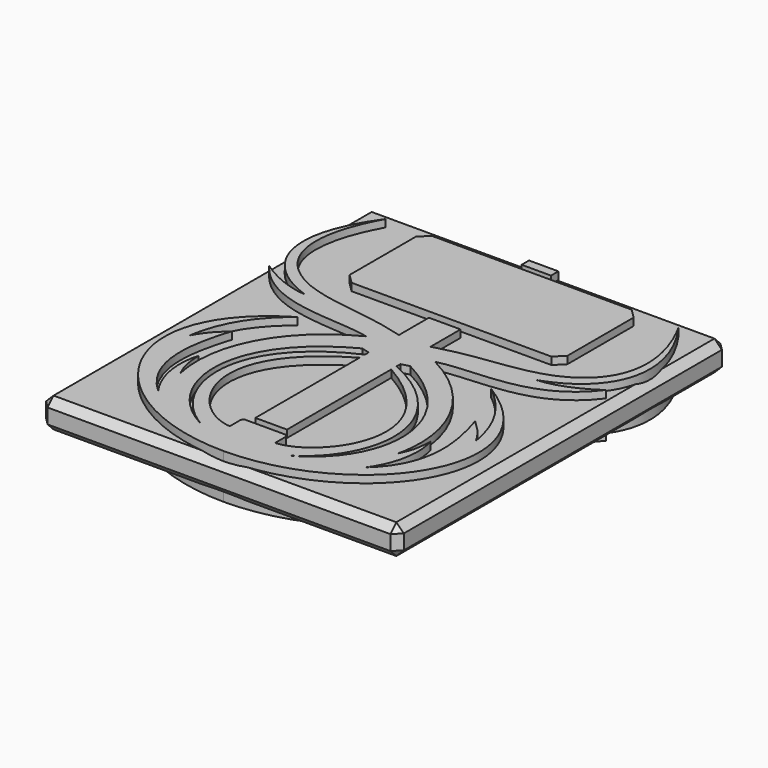
from build123d import *

# Parameters (mm, degrees)
F1_DEPTH     = 6.35
F2_DEPTH     = 9.525
F3_T1_DEPTH  = 4.0327916303
F3_T3_DEPTH  = 4.0327916303
F3_T5_DEPTH  = 4.0327916303
F3_T7_DEPTH  = 4.0327916303
F3_T9_DEPTH  = 4.0327916303
F3_T11_DEPTH = 4.0327916303
F3_T13_DEPTH = 4.0327916303
F3_T15_DEPTH = 4.0327916303
F3_T17_DEPTH = 29.0301869736
F3_T19_DEPTH = 192.1295719037
F3_T21_DEPTH = 168.7301869736


# Not quite as in the source:
# - a fillet or chamfer that OpenCascade refuses, or shapes differently, is made with other operations: its cross-section is extruded or revolved along the edge and cut away or added


with BuildPart() as f1:
    # F0 (on Top) → F1 (new body, symmetric)
    with BuildSketch(Plane.XY):
        Polygon((-76.3395167732, -75.9592950344), (-0.1395167732, -75.9592950344), (76.0604832268, -75.9592950344), (76.0604832268, 99.8400898957), (-0.3772020667, 99.8400898957), (-76.3395167732, 99.8400898957), align=None)
        with BuildLine():
            Line((-6.8799913861, 44.2892052233), (-0.1395167732, 44.2892052233))
            Line((-0.1395167732, 44.2892052233), (6.6009578396, 44.2892052233))
            Line((6.6009578396, 44.2892052233), (6.6009578396, 28.3039733768))
            add(Edge.make_bspline(
                [(6.6009578396, 28.3039733768), (26.5900306505, 33.9711308479), (37.0916825043, 32.1136220375), (51.7776187764, 37.7081698754)],
                knots=[0, 0, 0, 0, 46.1450929697, 46.1450929697, 46.1450929697, 46.1450929697], degree=3))
            add(Edge.make_bspline(
                [(51.7776187764, 37.7081698754), (73.0898510766, 46.7012859881), (75.5619611692, 66.6821375489), (62.3242836547, 90.7550230622)],
                knots=[0, 0, 0, 0, 54.0851252479, 54.0851252479, 54.0851252479, 54.0851252479], degree=3))
            add(Edge.make_bspline(
                [(62.3242836547, 90.7550230622), (70.2098065026, 79.8010850957), (73.6896972191, 69.8762632372), (73.6896974189, 61.3201553811)],
                knots=[0, 0, 0, 0, 22.7856930091, 22.7856930091, 22.7856930091, 22.7856930091], degree=3))
            add(Edge.make_bspline(
                [(73.6896974189, 61.3201553811), (73.6896977509, 47.1026080353), (64.0810465009, 36.6643450953), (49.1112602689, 31.5635202295)],
                knots=[22.7856930091, 22.7856930091, 22.7856930091, 22.7856930091, 60.6483140293, 60.6483140293, 60.6483140293, 60.6483140293], degree=3))
            add(Edge.make_bspline(
                [(49.1112602689, 31.5635202295), (56.512868042, 32.0529900491), (64.7170897674, 35.515807569), (71.6427248072, 40.4170304537)],
                knots=[0, 0, 0, 0, 24.2085013484, 24.2085013484, 24.2085013484, 24.2085013484], degree=3))
            add(Edge.make_bspline(
                [(71.6427248072, 40.4170304537), (55.7588432085, 19.1547237337), (30.2959364009, 24.5825536549), (14.5286014405, 20.7954701036)],
                knots=[0, 0, 0, 0, 60.390634361, 60.390634361, 60.390634361, 60.390634361], degree=3))
            add(Edge.make_bspline(
                [(14.5286014405, 20.7954701036), (41.5803175521, 6.7990645766), (51.0726925087, -18.260801211), (46.0924860191, -38.8492196798)],
                knots=[0, 0, 0, 0, 67.4816110437, 67.4816110437, 67.4816110437, 67.4816110437], degree=3))
            add(Edge.make_bspline(
                [(46.0924860191, -38.8492196798), (48.3534094047, -34.169908613), (49.0401517701, -31.6784828901), (49.3026469004, -25.0572301447)],
                knots=[0, 0, 0, 0, 14.1606535238, 14.1606535238, 14.1606535238, 14.1606535238], degree=3))
            add(Edge.make_bspline(
                [(49.3026469004, -25.0572301447), (51.7310705137, -32.9342447221), (50.7265012812, -43.7572076917), (44.0818425369, -53.0597306788)],
                knots=[0, 0, 0, 0, 28.4850282493, 28.4850282493, 28.4850282493, 28.4850282493], degree=3))
            add(Edge.make_bspline(
                [(44.0818425369, -53.0597306788), (60.305254544, -38.450088352), (56.4526263725, -19.4557197392), (51.6902711343, -4.2840936221)],
                knots=[0, 0, 0, 0, 49.3654834475, 49.3654834475, 49.3654834475, 49.3654834475], degree=3))
            add(Edge.make_bspline(
                [(51.6902711343, -4.2840936221), (54.9464095485, -7.2530964389), (58.2408178699, -10.4841506109), (60.8383324098, -15.4891163111)],
                knots=[0, 0, 0, 0, 14.465115228, 14.465115228, 14.465115228, 14.465115228], degree=3))
            add(Edge.make_bspline(
                [(60.8383324098, -15.4891163111), (58.5245881331, -1.1494335486), (51.5281986546, 9.0760597959), (41.0085301947, 17.3916071653)],
                knots=[0, 0, 0, 0, 38.3974352297, 38.3974352297, 38.3974352297, 38.3974352297], degree=3))
            add(Edge.make_bspline(
                [(41.0085301947, 17.3916071653), (94.1427406025, -14.5556982607), (57.5462374937, -73.1422898984), (-0.1395167732, -73.4192950344)],
                knots=[0, 0, 0, 0, 99.6984539881, 99.6984539881, 99.6984539881, 99.6984539881], degree=3))
            add(Edge.make_bspline(
                [(-41.2875637412, 17.3916071653), (-94.4217741489, -14.5556982607), (-57.8252710402, -73.1422898984), (-0.1395167732, -73.4192950344)],
                knots=[0, 0, 0, 0, 99.6984539881, 99.6984539881, 99.6984539881, 99.6984539881], degree=3))
            add(Edge.make_bspline(
                [(-61.1173659563, -15.4891163111), (-58.8036216795, -1.1494335486), (-51.8072322011, 9.0760597959), (-41.2875637412, 17.3916071653)],
                knots=[0, 0, 0, 0, 38.3974352297, 38.3974352297, 38.3974352297, 38.3974352297], degree=3))
            add(Edge.make_bspline(
                [(-51.9693046808, -4.2840936221), (-55.225443095, -7.2530964389), (-58.5198514163, -10.4841506109), (-61.1173659563, -15.4891163111)],
                knots=[0, 0, 0, 0, 14.465115228, 14.465115228, 14.465115228, 14.465115228], degree=3))
            add(Edge.make_bspline(
                [(-44.3608760834, -53.0597306788), (-60.5842880905, -38.450088352), (-56.731659919, -19.4557197392), (-51.9693046808, -4.2840936221)],
                knots=[0, 0, 0, 0, 49.3654834475, 49.3654834475, 49.3654834475, 49.3654834475], degree=3))
            add(Edge.make_bspline(
                [(-49.5816804469, -25.0572301447), (-52.0101040602, -32.9342447221), (-51.0055348277, -43.7572076917), (-44.3608760834, -53.0597306788)],
                knots=[0, 0, 0, 0, 28.4850282493, 28.4850282493, 28.4850282493, 28.4850282493], degree=3))
            add(Edge.make_bspline(
                [(-46.3715195656, -38.8492196798), (-48.6324429512, -34.169908613), (-49.3191853166, -31.6784828901), (-49.5816804469, -25.0572301447)],
                knots=[0, 0, 0, 0, 14.1606535238, 14.1606535238, 14.1606535238, 14.1606535238], degree=3))
            add(Edge.make_bspline(
                [(-14.8076349869, 20.7954701036), (-41.8593510985, 6.7990645766), (-51.3517260551, -18.260801211), (-46.3715195656, -38.8492196798)],
                knots=[0, 0, 0, 0, 67.4816110437, 67.4816110437, 67.4816110437, 67.4816110437], degree=3))
            add(Edge.make_bspline(
                [(-71.9217583537, 40.4170304537), (-56.037876755, 19.1547237337), (-30.5749699473, 24.5825536549), (-14.8076349869, 20.7954701036)],
                knots=[0, 0, 0, 0, 60.390634361, 60.390634361, 60.390634361, 60.390634361], degree=3))
            add(Edge.make_bspline(
                [(-49.3902938154, 31.5635202295), (-56.7919015884, 32.0529900491), (-64.9961233139, 35.515807569), (-71.9217583537, 40.4170304537)],
                knots=[0, 0, 0, 0, 24.2085013484, 24.2085013484, 24.2085013484, 24.2085013484], degree=3))
            add(Edge.make_bspline(
                [(-73.9687309654, 61.3201553811), (-73.9687312974, 47.1026080353), (-64.3600800474, 36.6643450953), (-49.3902938154, 31.5635202295)],
                knots=[22.7856930091, 22.7856930091, 22.7856930091, 22.7856930091, 60.6483140293, 60.6483140293, 60.6483140293, 60.6483140293], degree=3))
            add(Edge.make_bspline(
                [(-62.6033172011, 90.7550230622), (-70.4888400491, 79.8010850957), (-73.9687307656, 69.8762632372), (-73.9687309654, 61.3201553811)],
                knots=[0, 0, 0, 0, 22.7856930091, 22.7856930091, 22.7856930091, 22.7856930091], degree=3))
            add(Edge.make_bspline(
                [(-52.0566523229, 37.7081698754), (-73.3688846231, 46.7012859881), (-75.8409947157, 66.6821375489), (-62.6033172011, 90.7550230622)],
                knots=[0, 0, 0, 0, 54.0851252479, 54.0851252479, 54.0851252479, 54.0851252479], degree=3))
            add(Edge.make_bspline(
                [(-6.8799913861, 28.3039733768), (-26.8690641969, 33.9711308479), (-37.3707160507, 32.1136220375), (-52.0566523229, 37.7081698754)],
                knots=[0, 0, 0, 0, 46.1450929697, 46.1450929697, 46.1450929697, 46.1450929697], degree=3))
            Line((-6.8799913861, 28.3039733768), (-6.8799913861, 44.2892052233))
        make_face(mode=Mode.SUBTRACT)
        Polygon((-46.7502180452, 87.1615596313), (-42.9751879819, 90.9365896945), (42.2207838486, 90.9365896945), (46.2334992052, 86.9238743379), (46.2334992052, 51.6543717875), (42.458469142, 47.8793417243), (-42.7375026885, 47.8793417243), (-46.7502180452, 51.892057081), align=None, mode=Mode.SUBTRACT)
        Polygon((-6.6463192925, 97.3000898957), (-0.3772020667, 97.3000898957), (5.8919151591, 97.3000898957), (5.8919151591, 93.3534055948), (-0.3772020667, 93.3534055948), (-6.6463192925, 93.3534055948), align=None, mode=Mode.SUBTRACT)
    extrude(amount=F1_DEPTH, both=True)

    # F3: chamfer of 3.175 on 12 edges, made by hand

    # F3_s2 → F3_t1 (cut)
    with BuildSketch(Plane(origin=(50.6732594204, -50.6732594204, -50.6732594204), x_dir=(0.7071067812, 0.7071067812, 0), z_dir=(0.5773502692, -0.5773502692, -0.5773502692))):
        Polygon((0.071550857, 54.2846846585), (2.3166148873, 58.1732496251), (-2.1735131733, 58.1732496251), align=None)
    extrude(amount=F3_T1_DEPTH, mode=Mode.SUBTRACT)

    # F3_s4 → F3_t3 (cut)
    with BuildSketch(Plane(origin=(50.6732594204, -50.6732594204, 50.6732594204), x_dir=(0.7071067812, 0.7071067812, 0), z_dir=(0.5773502692, -0.5773502692, 0.5773502692))):
        Polygon((2.3166148873, -58.1732496251), (0.071550857, -54.2846846585), (-2.1735131733, -58.1732496251), align=None)
    extrude(amount=F3_T3_DEPTH, mode=Mode.SUBTRACT)

    # F3_s6 → F3_t5 (cut)
    with BuildSketch(Plane(origin=(58.6335243742, 58.6335243742, -58.6335243742), x_dir=(-0.7071067812, 0.7071067812, 0), z_dir=(0.5773502692, 0.5773502692, -0.5773502692))):
        Polygon((16.8147211296, 64.0339783355), (19.0597851598, 67.9225433022), (14.5696570993, 67.9225433022), align=None)
    extrude(amount=F3_T5_DEPTH, mode=Mode.SUBTRACT)

    # F3_s8 → F3_t7 (cut)
    with BuildSketch(Plane(origin=(58.6335243742, 58.6335243742, 58.6335243742), x_dir=(-0.7071067812, 0.7071067812, 0), z_dir=(0.5773502692, 0.5773502692, 0.5773502692))):
        Polygon((19.0597851598, -67.9225433022), (14.5696570993, -67.9225433022), (16.8147211296, -64.0339783355), align=None)
    extrude(amount=F3_T7_DEPTH, mode=Mode.SUBTRACT)

    # F3_s10 → F3_t9 (cut)
    with BuildSketch(Plane(origin=(-58.7265355563, 58.7265355563, -58.7265355563), x_dir=(-0.7071067812, -0.7071067812, 0), z_dir=(-0.5773502692, 0.5773502692, -0.5773502692))):
        Polygon((-14.3723505864, 68.0364582705), (-18.8624786469, 68.0364582705), (-16.6174146167, 64.1478933039), align=None)
    extrude(amount=F3_T9_DEPTH, mode=Mode.SUBTRACT)

    # F3_s12 → F3_t11 (cut)
    with BuildSketch(Plane(origin=(-50.7662706026, -50.7662706026, -50.7662706026), x_dir=(0.7071067812, -0.7071067812, 0), z_dir=(-0.5773502692, -0.5773502692, -0.5773502692))):
        Polygon((-2.5139214002, 58.2871645935), (-0.2688573699, 54.3985996268), (1.9762066604, 58.2871645935), align=None)
    extrude(amount=F3_T11_DEPTH, mode=Mode.SUBTRACT)

    # F3_s14 → F3_t13 (cut)
    with BuildSketch(Plane(origin=(-50.7662706026, -50.7662706026, 50.7662706026), x_dir=(0.7071067812, -0.7071067812, 0), z_dir=(-0.5773502692, -0.5773502692, 0.5773502692))):
        Polygon((-2.5139214002, -58.2871645935), (-0.2688573699, -54.3985996268), (1.9762066604, -58.2871645935), align=None)
    extrude(amount=F3_T13_DEPTH, mode=Mode.SUBTRACT)

    # F3_s16 → F3_t15 (cut)
    with BuildSketch(Plane(origin=(-58.7265355563, 58.7265355563, 58.7265355563), x_dir=(-0.7071067812, -0.7071067812, 0), z_dir=(-0.5773502692, 0.5773502692, 0.5773502692))):
        Polygon((-14.3723505864, -68.0364582705), (-18.8624786469, -68.0364582705), (-16.6174146167, -64.1478933039), align=None)
    extrude(amount=F3_T15_DEPTH, mode=Mode.SUBTRACT)

    # F3_s18 → F3_t17 (cut)
    with BuildSketch(Plane.XY.offset(-14.5150934868)):
        Polygon((76.0604832268, -72.7842950344), (72.8854832268, -75.9592950344), (76.0604832268, -75.9592950344), align=None)
        Polygon((72.8854832268, 99.8400898957), (76.0604832268, 96.6650898957), (76.0604832268, 99.8400898957), align=None)
        Polygon((-76.3395167732, -72.7842950344), (-73.1645167732, -75.9592950344), (-76.3395167732, -75.9592950344), align=None)
        Polygon((-76.3395167732, 96.6650898957), (-73.1645167732, 99.8400898957), (-76.3395167732, 99.8400898957), align=None)
    extrude(amount=F3_T17_DEPTH, mode=Mode.SUBTRACT)

    # F3_s20 → F3_t19 (cut)
    with BuildSketch(Plane.XZ.offset(-108.0051833825)):
        Polygon((76.0604832268, -3.175), (72.8854832268, -6.35), (76.0604832268, -6.35), align=None)
        Polygon((76.0604832268, 3.175), (72.8854832268, 6.35), (76.0604832268, 6.35), align=None)
        Polygon((-76.3395167732, -3.175), (-73.1645167732, -6.35), (-76.3395167732, -6.35), align=None)
        Polygon((-76.3395167732, 3.175), (-73.1645167732, 6.35), (-76.3395167732, 6.35), align=None)
    extrude(amount=F3_T19_DEPTH, mode=Mode.SUBTRACT)

    # F3_s22 → F3_t21 (cut)
    with BuildSketch(Plane.YZ.offset(-84.50461026)):
        Polygon((99.8400898957, 3.175), (96.6650898957, 6.35), (99.8400898957, 6.35), align=None)
        Polygon((99.8400898957, -3.175), (96.6650898957, -6.35), (99.8400898957, -6.35), align=None)
        Polygon((-75.9592950344, -3.175), (-72.7842950344, -6.35), (-75.9592950344, -6.35), align=None)
        Polygon((-72.7842950344, 6.35), (-75.9592950344, 3.175), (-75.9592950344, 6.35), align=None)
    extrude(amount=F3_T21_DEPTH, mode=Mode.SUBTRACT)


with BuildPart() as f1b:
    # F0 (on Top) → F1, piece 2 (new body, symmetric)
    with BuildSketch(Plane.XY):
        with BuildLine():
            Line((10.0785959613, 13.1602436304), (6.6009578396, 12.2357811779))
            Line((6.6009578396, 12.2357811779), (6.6009578396, 10.2524096146))
            add(Edge.make_bspline(
                [(6.6009578396, 10.2524096146), (49.2393244159, -9.3698259443), (42.5547603619, -48.4816730022), (18.2863567125, -62.6636892557)],
                knots=[0, 0, 0, 0, 73.8465031081, 73.8465031081, 73.8465031081, 73.8465031081], degree=3))
            add(Edge.make_bspline(
                [(10.0785959613, 13.1602436304), (50.5656320703, -8.0102328211), (46.5370509874, -48.0550006032), (18.2863567125, -62.6636892557)],
                knots=[0, 0, 0, 0, 76.266874427, 76.266874427, 76.266874427, 76.266874427], degree=3))
        make_face()
    extrude(amount=F1_DEPTH, both=True)


with BuildPart() as f1c:
    # F0 (on Top) → F1, piece 3 (new body, symmetric)
    with BuildSketch(Plane.XY):
        with BuildLine():
            Line((-6.8799913861, 10.2524096146), (-6.8799913861, 12.2357811779))
            Line((-6.8799913861, 12.2357811779), (-10.3576295078, 13.1602436304))
            add(Edge.make_bspline(
                [(-10.3576295078, 13.1602436304), (-50.8446656168, -8.0102328211), (-46.8160845339, -48.0550006032), (-18.565390259, -62.6636892557)],
                knots=[0, 0, 0, 0, 76.266874427, 76.266874427, 76.266874427, 76.266874427], degree=3))
            add(Edge.make_bspline(
                [(-6.8799913861, 10.2524096146), (-49.5183579624, -9.3698259443), (-42.8337939084, -48.4816730022), (-18.565390259, -62.6636892557)],
                knots=[0, 0, 0, 0, 73.8465031081, 73.8465031081, 73.8465031081, 73.8465031081], degree=3))
        make_face()
    extrude(amount=F1_DEPTH, both=True)


with BuildPart() as f1d:
    # F0 (on Top) → F1, piece 4 (new body, symmetric)
    with BuildSketch(Plane.XY):
        with BuildLine():
            Line((-6.8799913861, -48.1430366635), (-6.8799913861, 7.4029280804))
            add(Edge.make_bspline(
                [(-6.8799913861, 7.4029280804), (-54.2476996779, -19.9007634073), (-27.8019402176, -56.9516755641), (-9.7830155864, -58.1491813064)],
                knots=[0, 0, 0, 0, 65.6163591992, 65.6163591992, 65.6163591992, 65.6163591992], degree=3))
            Line((-9.7830155864, -58.1491813064), (-9.7830155864, -52.2294081748))
            Line((-9.7830155864, -52.2294081748), (-8.9240176603, -51.2886494398))
            Line((-8.9240176603, -51.2886494398), (-0.1395167732, -51.2886494398))
            Line((-0.1395167732, -51.2886494398), (8.6449841138, -51.2886494398))
            Line((8.6449841138, -51.2886494398), (9.5039820399, -52.2294081748))
            Line((9.5039820399, -52.2294081748), (9.5039820399, -58.1491813064))
            add(Edge.make_bspline(
                [(6.6009578396, 7.4029280804), (53.9686661315, -19.9007634073), (27.5229066711, -56.9516755641), (9.5039820399, -58.1491813064)],
                knots=[0, 0, 0, 0, 65.6163591992, 65.6163591992, 65.6163591992, 65.6163591992], degree=3))
            Line((6.6009578396, 7.4029280804), (6.6009578396, -48.1430366635))
            Line((6.6009578396, -48.1430366635), (-0.1395167732, -48.1430366635))
            Line((-0.1395167732, -48.1430366635), (-6.8799913861, -48.1430366635))
        make_face()
    extrude(amount=F1_DEPTH, both=True)


with BuildPart() as f2:
    # F0 (on Top) → F2 (new body, symmetric)
    with BuildSketch(Plane.XY):
        Polygon((42.2207838486, 90.9365896945), (-42.9751879819, 90.9365896945), (-46.7502180452, 87.1615596313), (-46.7502180452, 51.892057081), (-42.7375026885, 47.8793417243), (42.458469142, 47.8793417243), (46.2334992052, 51.6543717875), (46.2334992052, 86.9238743379), align=None)
    extrude(amount=F2_DEPTH, both=True)


with BuildPart() as f2b:
    # F0 (on Top) → F2, piece 2 (new body, symmetric)
    with BuildSketch(Plane.XY):
        Polygon((5.8919151591, 97.3000898957), (-0.3772020667, 97.3000898957), (-6.6463192925, 97.3000898957), (-6.6463192925, 93.3534055948), (-0.3772020667, 93.3534055948), (5.8919151591, 93.3534055948), align=None)
    extrude(amount=F2_DEPTH, both=True)


with BuildPart() as f2c:
    # F0 (on Top) → F2, piece 3 (new body, symmetric)
    with BuildSketch(Plane.XY):
        Polygon((6.6009578396, 44.2892052233), (-0.1395167732, 44.2892052233), (-6.8799913861, 44.2892052233), (-6.8799913861, 28.3039733768), (-6.8799913861, 12.2357811779), (-6.8799913861, 10.2524096146), (-6.8799913861, 7.4029280804), (-6.8799913861, -48.1430366635), (-0.1395167732, -48.1430366635), (6.6009578396, -48.1430366635), (6.6009578396, 7.4029280804), (6.6009578396, 10.2524096146), (6.6009578396, 12.2357811779), (6.6009578396, 28.3039733768), align=None)
        with BuildLine():
            Line((-6.8799913861, 12.2357811779), (-6.8799913861, 28.3039733768))
            add(Edge.make_bspline(
                [(-6.8799913861, 28.3039733768), (-26.8690641969, 33.9711308479), (-37.3707160507, 32.1136220375), (-52.0566523229, 37.7081698754)],
                knots=[0, 0, 0, 0, 46.1450929697, 46.1450929697, 46.1450929697, 46.1450929697], degree=3))
            add(Edge.make_bspline(
                [(-52.0566523229, 37.7081698754), (-73.3688846231, 46.7012859881), (-75.8409947157, 66.6821375489), (-62.6033172011, 90.7550230622)],
                knots=[0, 0, 0, 0, 54.0851252479, 54.0851252479, 54.0851252479, 54.0851252479], degree=3))
            add(Edge.make_bspline(
                [(-62.6033172011, 90.7550230622), (-70.4888400491, 79.8010850957), (-73.9687307656, 69.8762632372), (-73.9687309654, 61.3201553811)],
                knots=[0, 0, 0, 0, 22.7856930091, 22.7856930091, 22.7856930091, 22.7856930091], degree=3))
            add(Edge.make_bspline(
                [(-73.9687309654, 61.3201553811), (-73.9687312974, 47.1026080353), (-64.3600800474, 36.6643450953), (-49.3902938154, 31.5635202295)],
                knots=[22.7856930091, 22.7856930091, 22.7856930091, 22.7856930091, 60.6483140293, 60.6483140293, 60.6483140293, 60.6483140293], degree=3))
            add(Edge.make_bspline(
                [(-49.3902938154, 31.5635202295), (-56.7919015884, 32.0529900491), (-64.9961233139, 35.515807569), (-71.9217583537, 40.4170304537)],
                knots=[0, 0, 0, 0, 24.2085013484, 24.2085013484, 24.2085013484, 24.2085013484], degree=3))
            add(Edge.make_bspline(
                [(-71.9217583537, 40.4170304537), (-56.037876755, 19.1547237337), (-30.5749699473, 24.5825536549), (-14.8076349869, 20.7954701036)],
                knots=[0, 0, 0, 0, 60.390634361, 60.390634361, 60.390634361, 60.390634361], degree=3))
            add(Edge.make_bspline(
                [(-14.8076349869, 20.7954701036), (-41.8593510985, 6.7990645766), (-51.3517260551, -18.260801211), (-46.3715195656, -38.8492196798)],
                knots=[0, 0, 0, 0, 67.4816110437, 67.4816110437, 67.4816110437, 67.4816110437], degree=3))
            add(Edge.make_bspline(
                [(-46.3715195656, -38.8492196798), (-48.6324429512, -34.169908613), (-49.3191853166, -31.6784828901), (-49.5816804469, -25.0572301447)],
                knots=[0, 0, 0, 0, 14.1606535238, 14.1606535238, 14.1606535238, 14.1606535238], degree=3))
            add(Edge.make_bspline(
                [(-49.5816804469, -25.0572301447), (-52.0101040602, -32.9342447221), (-51.0055348277, -43.7572076917), (-44.3608760834, -53.0597306788)],
                knots=[0, 0, 0, 0, 28.4850282493, 28.4850282493, 28.4850282493, 28.4850282493], degree=3))
            add(Edge.make_bspline(
                [(-44.3608760834, -53.0597306788), (-60.5842880905, -38.450088352), (-56.731659919, -19.4557197392), (-51.9693046808, -4.2840936221)],
                knots=[0, 0, 0, 0, 49.3654834475, 49.3654834475, 49.3654834475, 49.3654834475], degree=3))
            add(Edge.make_bspline(
                [(-51.9693046808, -4.2840936221), (-55.225443095, -7.2530964389), (-58.5198514163, -10.4841506109), (-61.1173659563, -15.4891163111)],
                knots=[0, 0, 0, 0, 14.465115228, 14.465115228, 14.465115228, 14.465115228], degree=3))
            add(Edge.make_bspline(
                [(-61.1173659563, -15.4891163111), (-58.8036216795, -1.1494335486), (-51.8072322011, 9.0760597959), (-41.2875637412, 17.3916071653)],
                knots=[0, 0, 0, 0, 38.3974352297, 38.3974352297, 38.3974352297, 38.3974352297], degree=3))
            add(Edge.make_bspline(
                [(-41.2875637412, 17.3916071653), (-94.4217741489, -14.5556982607), (-57.8252710402, -73.1422898984), (-0.1395167732, -73.4192950344)],
                knots=[0, 0, 0, 0, 99.6984539881, 99.6984539881, 99.6984539881, 99.6984539881], degree=3))
            add(Edge.make_bspline(
                [(41.0085301947, 17.3916071653), (94.1427406025, -14.5556982607), (57.5462374937, -73.1422898984), (-0.1395167732, -73.4192950344)],
                knots=[0, 0, 0, 0, 99.6984539881, 99.6984539881, 99.6984539881, 99.6984539881], degree=3))
            add(Edge.make_bspline(
                [(60.8383324098, -15.4891163111), (58.5245881331, -1.1494335486), (51.5281986546, 9.0760597959), (41.0085301947, 17.3916071653)],
                knots=[0, 0, 0, 0, 38.3974352297, 38.3974352297, 38.3974352297, 38.3974352297], degree=3))
            add(Edge.make_bspline(
                [(51.6902711343, -4.2840936221), (54.9464095485, -7.2530964389), (58.2408178699, -10.4841506109), (60.8383324098, -15.4891163111)],
                knots=[0, 0, 0, 0, 14.465115228, 14.465115228, 14.465115228, 14.465115228], degree=3))
            add(Edge.make_bspline(
                [(44.0818425369, -53.0597306788), (60.305254544, -38.450088352), (56.4526263725, -19.4557197392), (51.6902711343, -4.2840936221)],
                knots=[0, 0, 0, 0, 49.3654834475, 49.3654834475, 49.3654834475, 49.3654834475], degree=3))
            add(Edge.make_bspline(
                [(49.3026469004, -25.0572301447), (51.7310705137, -32.9342447221), (50.7265012812, -43.7572076917), (44.0818425369, -53.0597306788)],
                knots=[0, 0, 0, 0, 28.4850282493, 28.4850282493, 28.4850282493, 28.4850282493], degree=3))
            add(Edge.make_bspline(
                [(46.0924860191, -38.8492196798), (48.3534094047, -34.169908613), (49.0401517701, -31.6784828901), (49.3026469004, -25.0572301447)],
                knots=[0, 0, 0, 0, 14.1606535238, 14.1606535238, 14.1606535238, 14.1606535238], degree=3))
            add(Edge.make_bspline(
                [(14.5286014405, 20.7954701036), (41.5803175521, 6.7990645766), (51.0726925087, -18.260801211), (46.0924860191, -38.8492196798)],
                knots=[0, 0, 0, 0, 67.4816110437, 67.4816110437, 67.4816110437, 67.4816110437], degree=3))
            add(Edge.make_bspline(
                [(71.6427248072, 40.4170304537), (55.7588432085, 19.1547237337), (30.2959364009, 24.5825536549), (14.5286014405, 20.7954701036)],
                knots=[0, 0, 0, 0, 60.390634361, 60.390634361, 60.390634361, 60.390634361], degree=3))
            add(Edge.make_bspline(
                [(49.1112602689, 31.5635202295), (56.512868042, 32.0529900491), (64.7170897674, 35.515807569), (71.6427248072, 40.4170304537)],
                knots=[0, 0, 0, 0, 24.2085013484, 24.2085013484, 24.2085013484, 24.2085013484], degree=3))
            add(Edge.make_bspline(
                [(73.6896974189, 61.3201553811), (73.6896977509, 47.1026080353), (64.0810465009, 36.6643450953), (49.1112602689, 31.5635202295)],
                knots=[22.7856930091, 22.7856930091, 22.7856930091, 22.7856930091, 60.6483140293, 60.6483140293, 60.6483140293, 60.6483140293], degree=3))
            add(Edge.make_bspline(
                [(62.3242836547, 90.7550230622), (70.2098065026, 79.8010850957), (73.6896972191, 69.8762632372), (73.6896974189, 61.3201553811)],
                knots=[0, 0, 0, 0, 22.7856930091, 22.7856930091, 22.7856930091, 22.7856930091], degree=3))
            add(Edge.make_bspline(
                [(51.7776187764, 37.7081698754), (73.0898510766, 46.7012859881), (75.5619611692, 66.6821375489), (62.3242836547, 90.7550230622)],
                knots=[0, 0, 0, 0, 54.0851252479, 54.0851252479, 54.0851252479, 54.0851252479], degree=3))
            add(Edge.make_bspline(
                [(6.6009578396, 28.3039733768), (26.5900306505, 33.9711308479), (37.0916825043, 32.1136220375), (51.7776187764, 37.7081698754)],
                knots=[0, 0, 0, 0, 46.1450929697, 46.1450929697, 46.1450929697, 46.1450929697], degree=3))
            Line((6.6009578396, 28.3039733768), (6.6009578396, 12.2357811779))
            Line((6.6009578396, 12.2357811779), (10.0785959613, 13.1602436304))
            add(Edge.make_bspline(
                [(10.0785959613, 13.1602436304), (50.5656320703, -8.0102328211), (46.5370509874, -48.0550006032), (18.2863567125, -62.6636892557)],
                knots=[0, 0, 0, 0, 76.266874427, 76.266874427, 76.266874427, 76.266874427], degree=3))
            add(Edge.make_bspline(
                [(6.6009578396, 10.2524096146), (49.2393244159, -9.3698259443), (42.5547603619, -48.4816730022), (18.2863567125, -62.6636892557)],
                knots=[0, 0, 0, 0, 73.8465031081, 73.8465031081, 73.8465031081, 73.8465031081], degree=3))
            Line((6.6009578396, 10.2524096146), (6.6009578396, 7.4029280804))
            add(Edge.make_bspline(
                [(6.6009578396, 7.4029280804), (53.9686661315, -19.9007634073), (27.5229066711, -56.9516755641), (9.5039820399, -58.1491813064)],
                knots=[0, 0, 0, 0, 65.6163591992, 65.6163591992, 65.6163591992, 65.6163591992], degree=3))
            Line((9.5039820399, -58.1491813064), (9.5039820399, -52.2294081748))
            Line((9.5039820399, -52.2294081748), (8.6449841138, -51.2886494398))
            Line((8.6449841138, -51.2886494398), (-0.1395167732, -51.2886494398))
            Line((-0.1395167732, -51.2886494398), (-8.9240176603, -51.2886494398))
            Line((-8.9240176603, -51.2886494398), (-9.7830155864, -52.2294081748))
            Line((-9.7830155864, -52.2294081748), (-9.7830155864, -58.1491813064))
            add(Edge.make_bspline(
                [(-6.8799913861, 7.4029280804), (-54.2476996779, -19.9007634073), (-27.8019402176, -56.9516755641), (-9.7830155864, -58.1491813064)],
                knots=[0, 0, 0, 0, 65.6163591992, 65.6163591992, 65.6163591992, 65.6163591992], degree=3))
            Line((-6.8799913861, 7.4029280804), (-6.8799913861, 10.2524096146))
            add(Edge.make_bspline(
                [(-6.8799913861, 10.2524096146), (-49.5183579624, -9.3698259443), (-42.8337939084, -48.4816730022), (-18.565390259, -62.6636892557)],
                knots=[0, 0, 0, 0, 73.8465031081, 73.8465031081, 73.8465031081, 73.8465031081], degree=3))
            add(Edge.make_bspline(
                [(-10.3576295078, 13.1602436304), (-50.8446656168, -8.0102328211), (-46.8160845339, -48.0550006032), (-18.565390259, -62.6636892557)],
                knots=[0, 0, 0, 0, 76.266874427, 76.266874427, 76.266874427, 76.266874427], degree=3))
            Line((-10.3576295078, 13.1602436304), (-6.8799913861, 12.2357811779))
        make_face()
    extrude(amount=F2_DEPTH, both=True)


solid = Compound([f1.part, f1b.part, f1c.part, f1d.part, f2.part, f2b.part, f2c.part])
